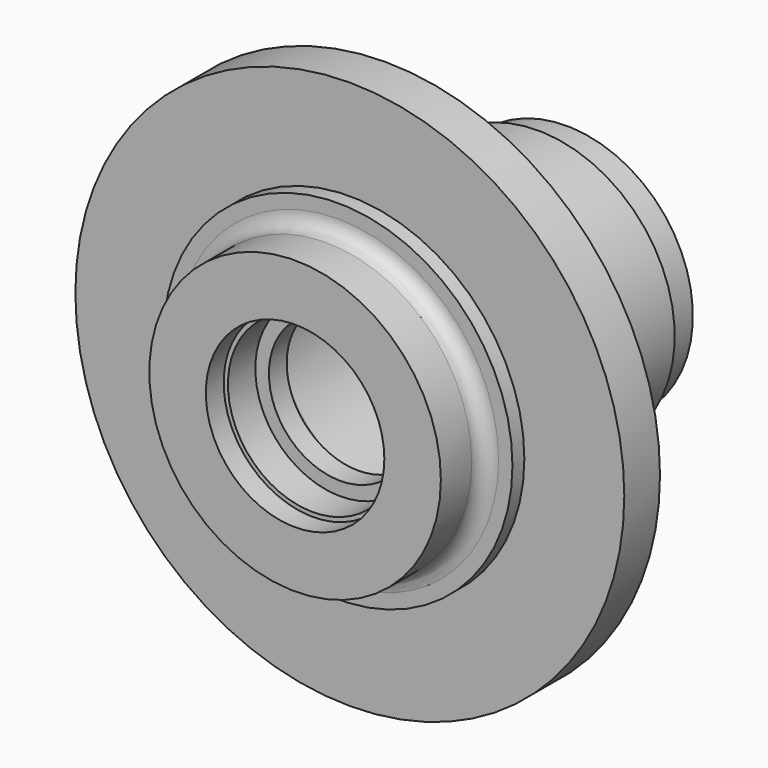
from build123d import *

# Parameters (mm, degrees)
F0_R      = 92.25
F1_DEPTH  = 114
F2_R      = 92.25
F2_R_2    = 49
F3_DEPTH  = 18
F4_R      = 5
F5_R      = 24
F6_DEPTH  = 26.5
F7_R      = 28.575
F8_DEPTH  = 19
F9_R      = 30
F10_DEPTH = 7.5
F11_R     = 92.25
F11_R_2   = 46
F12_DEPTH = 76
F13_R     = 46
F13_R_2   = 42.5
F14_DEPTH = 12
F15_R     = 31.5
F16_DEPTH = 42
F17_R     = 36.5125
F18_DEPTH = 32.5
F19_R     = 36
F20_DEPTH = 45.5
F21_R     = 11.99999
F22_R     = 5
F23_R     = 92.75
F23_R_2   = 58.66
F24_DEPTH = 23


# Not quite as in the source:
# - a fillet or chamfer is up to 0.001 mm smaller than in the source, because OpenCascade refuses the exact size


with BuildPart() as f1:
    # F0 (on Front) → F1 (new body)
    with BuildSketch(Plane.XZ):
        Circle(F0_R)
    extrude(amount=F1_DEPTH)

    # F2 (on face) → F3 (cut)
    with BuildSketch(Plane.XZ.offset(114)):
        Circle(F2_R)
        Circle(F2_R_2, mode=Mode.SUBTRACT)
    extrude(amount=-F3_DEPTH, mode=Mode.SUBTRACT)

    # F4
    f4_edges = [f1.edges().sort_by_distance(p)[0] for p in [
        (-49, -96, 0),
    ]]
    fillet(f4_edges, radius=F4_R)

    # F5 (on face) → F6 (cut)
    with BuildSketch(Plane.XZ.offset(114)):
        Circle(F5_R)
    extrude(amount=-F6_DEPTH, mode=Mode.SUBTRACT)

    # F7 (on face) → F8 (cut)
    with BuildSketch(Plane.XZ.offset(114)):
        Circle(F7_R)
    extrude(amount=-F8_DEPTH, mode=Mode.SUBTRACT)

    # F9 (on face) → F10 (cut)
    with BuildSketch(Plane.XZ.offset(114)):
        Circle(F9_R)
    extrude(amount=-F10_DEPTH, mode=Mode.SUBTRACT)

    # F11 (on face) → F12 (cut)
    with BuildSketch(Plane(origin=(0, 0, 0), x_dir=(-1, 0, 0), z_dir=(0, 1, 0))):
        Circle(F11_R)
        Circle(F11_R_2, mode=Mode.SUBTRACT)
    extrude(amount=-F12_DEPTH, mode=Mode.SUBTRACT)

    # F13 (on face) → F14 (cut)
    with BuildSketch(Plane(origin=(0, 0, 0), x_dir=(-1, 0, 0), z_dir=(0, 1, 0))):
        Circle(F13_R)
        Circle(F13_R_2, mode=Mode.SUBTRACT)
    extrude(amount=-F14_DEPTH, mode=Mode.SUBTRACT)

    # F15 (on face) → F16 (cut)
    with BuildSketch(Plane(origin=(0, 0, 0), x_dir=(-1, 0, 0), z_dir=(0, 1, 0))):
        Circle(F15_R)
    extrude(amount=-F16_DEPTH, mode=Mode.SUBTRACT)

    # F17 (on face) → F18 (cut)
    with BuildSketch(Plane(origin=(0, 0, 0), x_dir=(-1, 0, 0), z_dir=(0, 1, 0))):
        Circle(F17_R)
    extrude(amount=-F18_DEPTH, mode=Mode.SUBTRACT)

    # F19 (on face) → F20 (cut)
    with BuildSketch(Plane(origin=(0, -42, 0), x_dir=(-1, 0, 0), z_dir=(0, 1, 0))):
        Circle(F19_R)
    extrude(amount=-F20_DEPTH, mode=Mode.SUBTRACT)

    # F21 (radius 12 in the source; OpenCascade refuses exactly that, so slightly less here)
    f21_edges = [f1.edges().sort_by_distance(p)[0] for p in [
        (36, -87.5, 0),
    ]]
    fillet(f21_edges, radius=F21_R)

    # F22
    f22_edges = [f1.edges().sort_by_distance(p)[0] for p in [
        (46, -76, 0),
    ]]
    fillet(f22_edges, radius=F22_R)

    # F23 (on face) → F24 (cut)
    with BuildSketch(Plane.XZ.offset(114)):
        Circle(F23_R)
        Circle(F23_R_2, mode=Mode.SUBTRACT)
    extrude(amount=-F24_DEPTH, mode=Mode.SUBTRACT)


solid = f1.part
